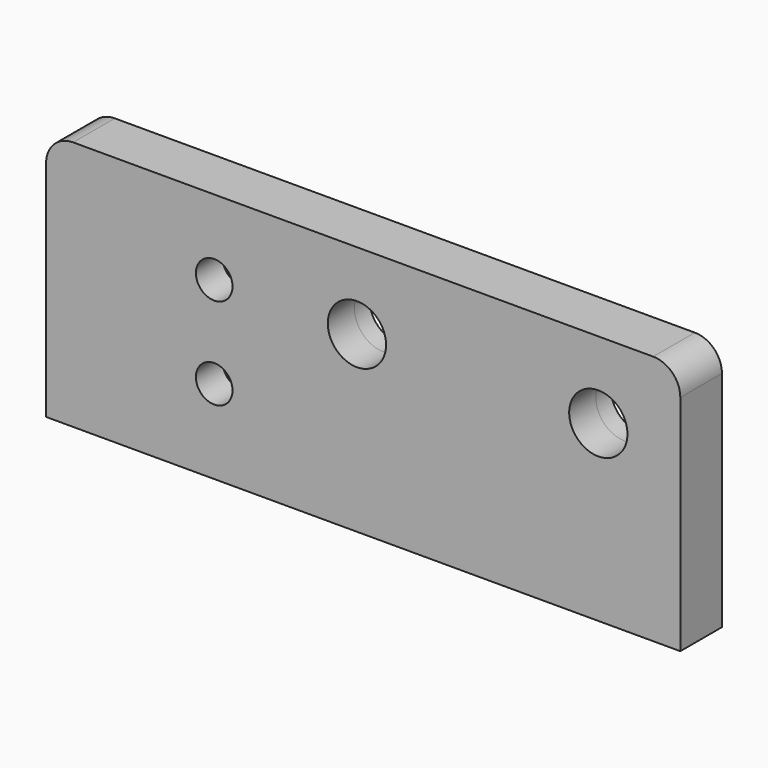
from build123d import *

# Parameters (mm, degrees)
F0_R     = 2.2
F0_R_2   = 3.5
F1_DEPTH = 4
F2_DEPTH = 2.251


with BuildPart() as f1:
    # F0 (on Front) → F1 (new body)
    with BuildSketch(Plane.XZ):
        with BuildLine():
            Line((-38.1, 26.8488), (-38.1, 0))
            Line((-38.1, 0), (38.1, 0))
            Line((38.1, 0), (38.1, 26.8488))
            ThreePointArc((38.1, 26.8488), (37.147745567, 29.147745567), (34.8488, 30.1))
            Line((34.8488, 30.1), (-34.8488, 30.1))
            ThreePointArc((-34.8488, 30.1), (-37.147745567, 29.147745567), (-38.1, 26.8488))
        make_face()
        with BuildLine():
            Line((-34.8488, 26.8488), (-4.245966041, 26.8488))
            ThreePointArc((-4.245966041, 26.8488), (-0.75, 27.8), (2.745966041, 26.8488))
            Line((2.745966041, 26.8488), (24.754033959, 26.8488))
            ThreePointArc((24.754033959, 26.8488), (28.25, 27.8), (31.745966041, 26.8488))
            Line((31.745966041, 26.8488), (34.8488, 26.8488))
            Line((34.8488, 26.8488), (34.8488, 22.9163924618))
            ThreePointArc((34.8488, 22.9163924618), (35.0742845779, 21.9193821658), (35.15, 20.9))
            ThreePointArc((35.15, 20.9), (35.0742845779, 19.8806178342), (34.8488, 18.8836075382))
            Line((34.8488, 18.8836075382), (34.8488, 3.2512))
            Line((34.8488, 3.2512), (29.8756, 3.2512))
            Line((29.8756, 3.2512), (26.6244, 3.2512))
            Line((26.6244, 3.2512), (0.8756, 3.2512))
            Line((0.8756, 3.2512), (-2.3756, 3.2512))
            Line((-2.3756, 3.2512), (-34.8488, 3.2512))
            Line((-34.8488, 3.2512), (-34.8488, 26.8488))
        make_face(mode=Mode.SUBTRACT)
        with BuildLine():
            Line((-2.3756, 3.2512), (-2.3756, 14.194224531))
            ThreePointArc((-2.3756, 14.194224531), (-7.5758464496, 19.8911292219), (-4.245966041, 26.8488))
            Line((-4.245966041, 26.8488), (-34.8488, 26.8488))
            Line((-34.8488, 26.8488), (-34.8488, 3.2512))
            Line((-34.8488, 3.2512), (-2.3756, 3.2512))
        make_face()
        with Locations((-17.9, 10.074)):
            Circle(F0_R, mode=Mode.SUBTRACT)
        with Locations((-17.9, 21.074)):
            Circle(F0_R, mode=Mode.SUBTRACT)
        with BuildLine():
            ThreePointArc((6.15, 20.9), (4.6734048346, 16.6342433262), (0.8756, 14.194224531))
            Line((0.8756, 14.194224531), (0.8756, 3.2512))
            Line((0.8756, 3.2512), (26.6244, 3.2512))
            Line((26.6244, 3.2512), (26.6244, 14.194224531))
            ThreePointArc((26.6244, 14.194224531), (21.4241535504, 19.8911292219), (24.754033959, 26.8488))
            Line((24.754033959, 26.8488), (2.745966041, 26.8488))
            ThreePointArc((2.745966041, 26.8488), (5.2388298391, 24.3269399117), (6.15, 20.9))
        make_face()
        with BuildLine():
            ThreePointArc((-4.245966041, 26.8488), (-7.5758464496, 19.8911292219), (-2.3756, 14.194224531))
            ThreePointArc((-2.3756, 14.194224531), (-0.75, 14), (0.8756, 14.194224531))
            ThreePointArc((0.8756, 14.194224531), (4.6734048346, 16.6342433262), (6.15, 20.9))
            ThreePointArc((6.15, 20.9), (5.2388298391, 24.3269399117), (2.745966041, 26.8488))
            Line((2.745966041, 26.8488), (-4.245966041, 26.8488))
        make_face()
        with Locations((-0.75, 20.9)):
            Circle(F0_R_2, mode=Mode.SUBTRACT)
        with BuildLine():
            Line((31.745966041, 26.8488), (24.754033959, 26.8488))
            ThreePointArc((24.754033959, 26.8488), (21.4241535504, 19.8911292219), (26.6244, 14.194224531))
            ThreePointArc((26.6244, 14.194224531), (28.25, 14), (29.8756, 14.194224531))
            ThreePointArc((29.8756, 14.194224531), (32.9836843037, 15.8798174423), (34.8488, 18.8836075382))
            Line((34.8488, 18.8836075382), (34.8488, 22.9163924618))
            ThreePointArc((34.8488, 22.9163924618), (33.6668286494, 25.1741042784), (31.745966041, 26.8488))
        make_face()
        with Locations((28.25, 20.9)):
            Circle(F0_R_2, mode=Mode.SUBTRACT)
        with BuildLine():
            Line((29.8756, 14.194224531), (29.8756, 3.2512))
            Line((29.8756, 3.2512), (34.8488, 3.2512))
            Line((34.8488, 3.2512), (34.8488, 18.8836075382))
            ThreePointArc((34.8488, 18.8836075382), (32.9836843037, 15.8798174423), (29.8756, 14.194224531))
        make_face()
        with BuildLine():
            Line((26.6244, 14.194224531), (26.6244, 3.2512))
            Line((26.6244, 3.2512), (29.8756, 3.2512))
            Line((29.8756, 3.2512), (29.8756, 14.194224531))
            ThreePointArc((29.8756, 14.194224531), (28.25, 14), (26.6244, 14.194224531))
        make_face()
        with BuildLine():
            ThreePointArc((0.8756, 14.194224531), (-0.75, 14), (-2.3756, 14.194224531))
            Line((-2.3756, 14.194224531), (-2.3756, 3.2512))
            Line((-2.3756, 3.2512), (0.8756, 3.2512))
            Line((0.8756, 3.2512), (0.8756, 14.194224531))
        make_face()
        with BuildLine():
            Line((34.8488, 26.8488), (31.745966041, 26.8488))
            ThreePointArc((31.745966041, 26.8488), (33.6668286494, 25.1741042784), (34.8488, 22.9163924618))
            Line((34.8488, 22.9163924618), (34.8488, 26.8488))
        make_face()
        with BuildLine():
            ThreePointArc((31.745966041, 26.8488), (28.25, 27.8), (24.754033959, 26.8488))
            Line((24.754033959, 26.8488), (31.745966041, 26.8488))
        make_face()
        with BuildLine():
            ThreePointArc((2.745966041, 26.8488), (-0.75, 27.8), (-4.245966041, 26.8488))
            Line((-4.245966041, 26.8488), (2.745966041, 26.8488))
        make_face()
        with BuildLine():
            ThreePointArc((35.15, 20.9), (35.0742845779, 21.9193821658), (34.8488, 22.9163924618))
            Line((34.8488, 22.9163924618), (34.8488, 18.8836075382))
            ThreePointArc((34.8488, 18.8836075382), (35.0742845779, 19.8806178342), (35.15, 20.9))
        make_face()
    extrude(amount=F1_DEPTH)

    # F0 (on Front) → F2 (join)
    with BuildSketch(Plane.XZ):
        with BuildLine():
            Line((-38.1, 26.8488), (-38.1, 0))
            Line((-38.1, 0), (38.1, 0))
            Line((38.1, 0), (38.1, 26.8488))
            ThreePointArc((38.1, 26.8488), (37.147745567, 29.147745567), (34.8488, 30.1))
            Line((34.8488, 30.1), (-34.8488, 30.1))
            ThreePointArc((-34.8488, 30.1), (-37.147745567, 29.147745567), (-38.1, 26.8488))
        make_face()
        with BuildLine():
            Line((-34.8488, 26.8488), (-4.245966041, 26.8488))
            ThreePointArc((-4.245966041, 26.8488), (-0.75, 27.8), (2.745966041, 26.8488))
            Line((2.745966041, 26.8488), (24.754033959, 26.8488))
            ThreePointArc((24.754033959, 26.8488), (28.25, 27.8), (31.745966041, 26.8488))
            Line((31.745966041, 26.8488), (34.8488, 26.8488))
            Line((34.8488, 26.8488), (34.8488, 22.9163924618))
            ThreePointArc((34.8488, 22.9163924618), (35.0742845779, 21.9193821658), (35.15, 20.9))
            ThreePointArc((35.15, 20.9), (35.0742845779, 19.8806178342), (34.8488, 18.8836075382))
            Line((34.8488, 18.8836075382), (34.8488, 3.2512))
            Line((34.8488, 3.2512), (29.8756, 3.2512))
            Line((29.8756, 3.2512), (26.6244, 3.2512))
            Line((26.6244, 3.2512), (0.8756, 3.2512))
            Line((0.8756, 3.2512), (-2.3756, 3.2512))
            Line((-2.3756, 3.2512), (-34.8488, 3.2512))
            Line((-34.8488, 3.2512), (-34.8488, 26.8488))
        make_face(mode=Mode.SUBTRACT)
        with BuildLine():
            ThreePointArc((-4.245966041, 26.8488), (-7.5758464496, 19.8911292219), (-2.3756, 14.194224531))
            ThreePointArc((-2.3756, 14.194224531), (-0.75, 14), (0.8756, 14.194224531))
            ThreePointArc((0.8756, 14.194224531), (4.6734048346, 16.6342433262), (6.15, 20.9))
            ThreePointArc((6.15, 20.9), (5.2388298391, 24.3269399117), (2.745966041, 26.8488))
            Line((2.745966041, 26.8488), (-4.245966041, 26.8488))
        make_face()
        with Locations((-0.75, 20.9)):
            Circle(F0_R_2, mode=Mode.SUBTRACT)
        with BuildLine():
            ThreePointArc((0.8756, 14.194224531), (-0.75, 14), (-2.3756, 14.194224531))
            Line((-2.3756, 14.194224531), (-2.3756, 3.2512))
            Line((-2.3756, 3.2512), (0.8756, 3.2512))
            Line((0.8756, 3.2512), (0.8756, 14.194224531))
        make_face()
        with BuildLine():
            ThreePointArc((2.745966041, 26.8488), (-0.75, 27.8), (-4.245966041, 26.8488))
            Line((-4.245966041, 26.8488), (2.745966041, 26.8488))
        make_face()
        with BuildLine():
            Line((26.6244, 14.194224531), (26.6244, 3.2512))
            Line((26.6244, 3.2512), (29.8756, 3.2512))
            Line((29.8756, 3.2512), (29.8756, 14.194224531))
            ThreePointArc((29.8756, 14.194224531), (28.25, 14), (26.6244, 14.194224531))
        make_face()
        with BuildLine():
            Line((31.745966041, 26.8488), (24.754033959, 26.8488))
            ThreePointArc((24.754033959, 26.8488), (21.4241535504, 19.8911292219), (26.6244, 14.194224531))
            ThreePointArc((26.6244, 14.194224531), (28.25, 14), (29.8756, 14.194224531))
            ThreePointArc((29.8756, 14.194224531), (32.9836843037, 15.8798174423), (34.8488, 18.8836075382))
            Line((34.8488, 18.8836075382), (34.8488, 22.9163924618))
            ThreePointArc((34.8488, 22.9163924618), (33.6668286494, 25.1741042784), (31.745966041, 26.8488))
        make_face()
        with Locations((28.25, 20.9)):
            Circle(F0_R_2, mode=Mode.SUBTRACT)
        with BuildLine():
            ThreePointArc((31.745966041, 26.8488), (28.25, 27.8), (24.754033959, 26.8488))
            Line((24.754033959, 26.8488), (31.745966041, 26.8488))
        make_face()
        with BuildLine():
            Line((34.8488, 26.8488), (31.745966041, 26.8488))
            ThreePointArc((31.745966041, 26.8488), (33.6668286494, 25.1741042784), (34.8488, 22.9163924618))
            Line((34.8488, 22.9163924618), (34.8488, 26.8488))
        make_face()
        with BuildLine():
            ThreePointArc((35.15, 20.9), (35.0742845779, 21.9193821658), (34.8488, 22.9163924618))
            Line((34.8488, 22.9163924618), (34.8488, 18.8836075382))
            ThreePointArc((34.8488, 18.8836075382), (35.0742845779, 19.8806178342), (35.15, 20.9))
        make_face()
    extrude(amount=-F2_DEPTH)


solid = f1.part
